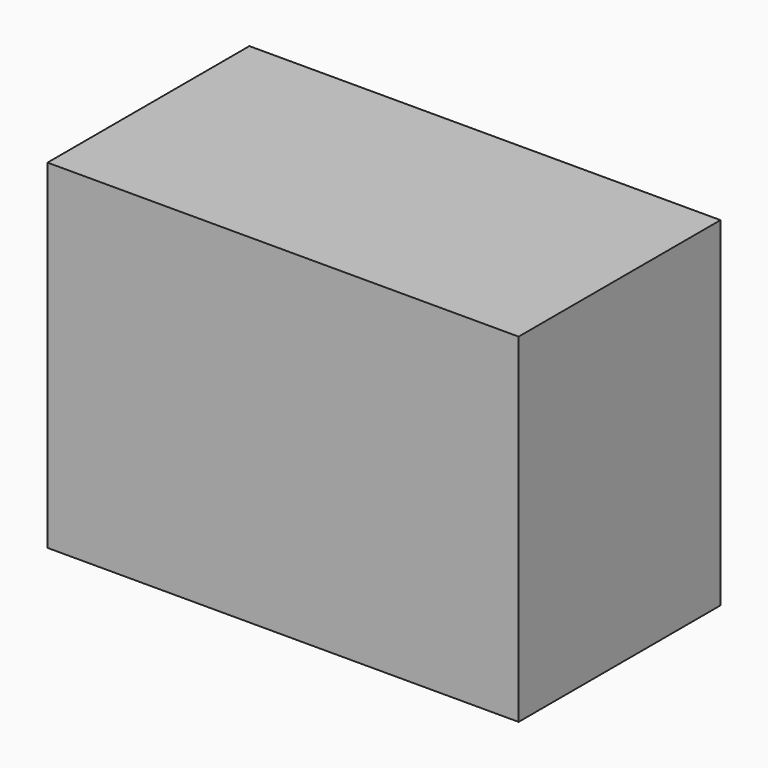
from build123d import *

# Parameters (mm, degrees)
F1_W     = 5000
F1_H     = 3600
F2_DEPTH = 2677.9042482376


# Not quite as in the source:
# - the program builds the solid bodies; features that only make, move or delete a surface that nothing else refers to are left out


with BuildPart() as f2:
    # F1 (on face) → F2 (new body)
    with BuildSketch(Plane.XZ):
        with Locations((887.5499308877, 25.326564908)):
            Rectangle(F1_W, F1_H)
    extrude(amount=F2_DEPTH)


solid = f2.part
